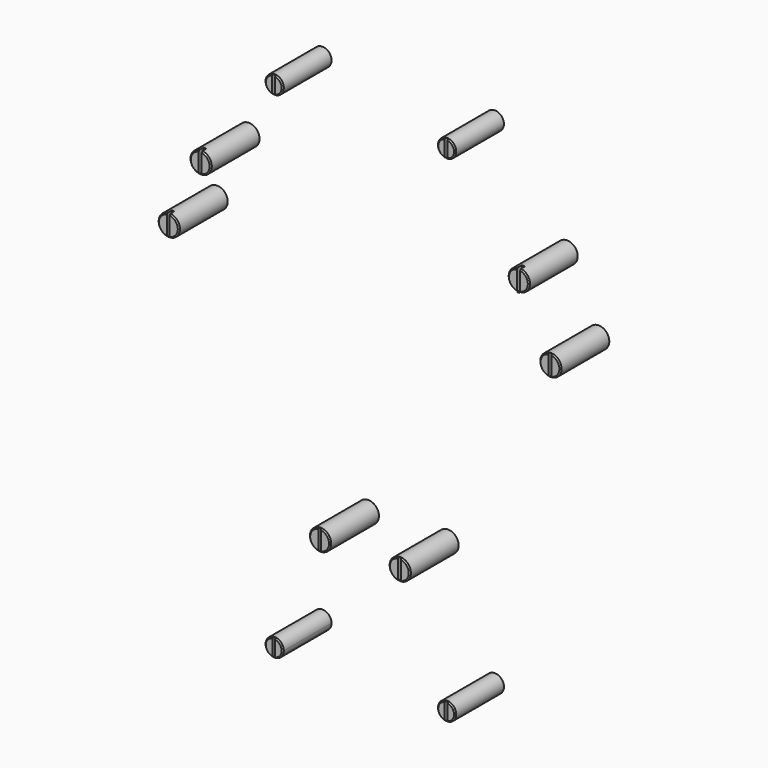
from build123d import *

# Parameters (mm, degrees)
F2_DEPTH      = 25.4
F0_R          = 3.81
F1_R          = 4.445
F4_START      = 22.86
F3_W          = 1.2230351567
F3_H          = 8.8948234916
F3_W_2        = 1.1118501425
F3_W_3        = 1.334220171
F3_H_2        = 8.78364034
F3_W_4        = 1.2230370194
F3_H_3        = 8.5612684488
F3_W_5        = 1.0006669909
F3_H_4        = 8.6724534631
F3_W_6        = 1.0006688535
F3_H_5        = 7.2270408273
F3_W_7        = 1.223038882
F3_W_8        = 1.2295618653
F3_H_6        = 7.377371192
F3_W_9        = 1.3241432607
F3_H_7        = 7.4719488621
F4_DEPTH      = 23.114
F5_4_T2_ANGLE = 279.074624531
F5_4_T4_ANGLE = 119.2903176817
F5_7_C1_SIZE  = 0.508
F5_7_C2_SIZE  = 0.508
F5_8_T2_ANGLE = 278.1597188723
F5_8_T4_ANGLE = 99.7656947124
F5_9_C1_SIZE  = 0.508
F5_9_C2_SIZE  = 0.508


# Not quite as in the source:
# - a fillet or chamfer that OpenCascade refuses, or shapes differently, is made with other operations: its cross-section is extruded or revolved along the edge and cut away or added


with BuildPart() as f2:
    # F0 (on Front) → F2 (new body)
    with BuildSketch(Plane.XZ):
        with BuildLine():
            ThreePointArc((-39.431919848, -111.8159154973), (-35.5624732541, -115.5025815711), (-31.8139005923, -111.6930767894))
            ThreePointArc((-31.8139005923, -111.6930767894), (-35.6853279305, -107.8835720076), (-39.431919848, -111.8159154973))
        make_face()
    extrude(amount=F2_DEPTH)


with BuildPart() as f2b:
    # F0 (on Front) → F2, piece 2 (new body)
    with BuildSketch(Plane.XZ):
        with Locations((36.3284870982, -111.6930693388)):
            Circle(F0_R)
    extrude(amount=F2_DEPTH)


with BuildPart() as f2c:
    # F0 (on Front) → F2, piece 3 (new body)
    with BuildSketch(Plane.XZ):
        with Locations((-35.6239005923, 95.0886905193)):
            Circle(F0_R)
    extrude(amount=F2_DEPTH)


with BuildPart() as f2d:
    # F0 (on Front) → F2, piece 4 (new body)
    with BuildSketch(Plane.XZ):
        with Locations((36.3284870982, 95.0886905193)):
            Circle(F0_R)
    extrude(amount=F2_DEPTH)


with BuildPart() as f2e:
    # F1 (on Front) → F2, piece 5 (new body)
    with BuildSketch(Plane.XZ):
        with Locations((16.7914066574, -65.8985787277)):
            Circle(F1_R)
    extrude(amount=F2_DEPTH)


with BuildPart() as f2f:
    # F1 (on Front) → F2, piece 6 (new body)
    with BuildSketch(Plane.XZ):
        with Locations((-16.4702718891, -65.8985787277)):
            Circle(F1_R)
    extrude(amount=F2_DEPTH)


with BuildPart() as f2g:
    # F1 (on Front) → F2, piece 7 (new body)
    with BuildSketch(Plane.XZ):
        with Locations((-79.6014981537, 29.1146653051)):
            Circle(F1_R)
    extrude(amount=F2_DEPTH)


with BuildPart() as f2h:
    # F1 (on Front) → F2, piece 8 (new body)
    with BuildSketch(Plane.XZ):
        with Locations((-66.3161736801, 56.4890627044)):
            Circle(F1_R)
    extrude(amount=F2_DEPTH)


with BuildPart() as f2i:
    # F1 (on Front) → F2, piece 9 (new body)
    with BuildSketch(Plane.XZ):
        with Locations((66.4782037265, 56.4889616946)):
            Circle(F1_R)
    extrude(amount=F2_DEPTH)


with BuildPart() as f2j:
    # F1 (on Front) → F2, piece 10 (new body)
    with BuildSketch(Plane.XZ):
        with Locations((79.6604069033, 29.5357785845)):
            Circle(F1_R)
    extrude(amount=F2_DEPTH)


with BuildPart() as f4_tool:
    # F3 (on Front) → F4 (new body)
    with BuildSketch(Plane.XZ.offset(F4_START)):
        with Locations((-66.3798488677, 56.613355875)):
            Rectangle(F3_W, F3_H)
        with Locations((-79.6664953232, 29.1505865753)):
            Rectangle(F3_W_2, F3_H)
        with Locations((66.5421783924, 56.5021708608)):
            Rectangle(F3_W_3, F3_H)
        with Locations((79.6620473266, 29.5397331938)):
            Rectangle(F3_W_2, F3_H_2)
        with Locations((16.7867569253, -65.8572539687)):
            Rectangle(F3_W_4, F3_H_3)
        with Locations((-16.4576480165, -65.9128464758)):
            Rectangle(F3_W_5, F3_H_4)
        with Locations((-35.5815198272, -111.6655953228)):
            Rectangle(F3_W_6, F3_H_5)
        with Locations((36.3553669304, -111.7767803371)):
            Rectangle(F3_W_7, F3_H_5)
        with Locations((-35.6421023607, 95.0211137533)):
            Rectangle(F3_W_8, F3_H_6)
        with Locations((36.2872686237, 95.0684025884)):
            Rectangle(F3_W_9, F3_H_7)
    extrude(amount=F4_DEPTH)


with BuildPart() as f2_1:
    add(f2.part)

    # F4: cut by f4_tool
    add(f4_tool.part, mode=Mode.SUBTRACT)

    # F5: chamfer of 0.508 on 1 edges, made by hand

    # F5_s1 → F5_t2 (revolve, cut)
    with BuildSketch(Plane(origin=(3.5622082334, 0, -110.4290151723), x_dir=(0, 1, 0), z_dir=(0.0322411307, 0, -0.9994801196))):
        Polygon((-24.892, -43.016491512), (-25.4, -42.508491512), (-25.4, -43.016491512), align=None)
    revolve(axis=Axis((-35.6239005923, -25.4, -111.6930767894), (0, 1, 0)), mode=Mode.SUBTRACT)


with BuildPart() as f2b_1:
    add(f2b.part)

    # F4: cut by f4_tool
    add(f4_tool.part, mode=Mode.SUBTRACT)

    # F5#2: chamfer of 0.508 on 1 edges, made by hand

    # F5_2_s1 → F5_2_t2 (revolve, cut)
    with BuildSketch(Plane.XY.offset(-111.6930693388)):
        Polygon((40.1384870982, -24.892), (39.6304870982, -25.4), (40.1384870982, -25.4), align=None)
    revolve(axis=Axis((36.3284870982, -25.4, -111.6930693388), (0, -1, 0)), mode=Mode.SUBTRACT)


with BuildPart() as f2c_1:
    add(f2c.part)

    # F4: cut by f4_tool
    add(f4_tool.part, mode=Mode.SUBTRACT)

    # F5#3: chamfer of 0.508 on 1 edges, made by hand

    # F5_3_s1 → F5_3_t2 (revolve, cut)
    with BuildSketch(Plane.XY.offset(95.0886905193)):
        Polygon((-31.8139005923, -24.892), (-32.3219005923, -25.4), (-31.8139005923, -25.4), align=None)
    revolve(axis=Axis((-35.6239005923, -25.4, 95.0886905193), (0, -1, 0)), mode=Mode.SUBTRACT)


with BuildPart() as f2d_1:
    add(f2d.part)

    # F4: cut by f4_tool
    add(f4_tool.part, mode=Mode.SUBTRACT)

    # F5#4: chamfer of 0.508 on 2 edges, made by hand

    # F5_4_s1 → F5_4_t2 (revolve, cut)
    with BuildSketch(Plane.XY.offset(95.0886905193)):
        with BuildLine():
            Line((40.152855508, -24.8776315902), (39.6161186884, -25.4143684098))
            Line((39.6161186884, -25.4143684098), (39.6161186884, -25.4245284098))
            ThreePointArc((39.6161186884, -25.4245284098), (39.8773028933, -25.41016), (40.1384870982, -25.41016))
            Line((40.1384870982, -25.41016), (40.1486470982, -25.4))
            ThreePointArc((40.1486470982, -25.4), (40.1486470982, -25.1388157951), (40.163015508, -24.8776315902))
            Line((40.163015508, -24.8776315902), (40.152855508, -24.8776315902))
        make_face()
    revolve(axis=Axis((36.3284870982, -25.4, 95.0886905193), (0, -1, 0)), revolution_arc=F5_4_T2_ANGLE, mode=Mode.SUBTRACT)

    # F5_4_s3 → F5_4_t4 (revolve, cut)
    with BuildSketch(Plane(origin=(-12.9399105656, 0, 7.2586640976), x_dir=(0, 1, 0), z_dir=(-0.8721519599, 0, 0.4892350752))):
        with BuildLine():
            Line((-24.8776315902, -96.8805895099), (-25.4143684098, -97.4173263294))
            Line((-25.4143684098, -97.4173263294), (-25.4245284098, -97.4173263294))
            ThreePointArc((-25.4245284098, -97.4173263294), (-25.41016, -97.1561421246), (-25.41016, -96.8949579197))
            Line((-25.41016, -96.8949579197), (-25.4, -96.8847979197))
            ThreePointArc((-25.4, -96.8847979197), (-25.1388157951, -96.8847979197), (-24.8776315902, -96.8704295099))
            Line((-24.8776315902, -96.8704295099), (-24.8776315902, -96.8805895099))
        make_face()
    revolve(axis=Axis((36.3284870982, -25.4, 95.0886905193), (0, -1, 0)), revolution_arc=F5_4_T4_ANGLE, mode=Mode.SUBTRACT)


with BuildPart() as f2e_1:
    add(f2e.part)

    # F4: cut by f4_tool
    add(f4_tool.part, mode=Mode.SUBTRACT)

    # F5#5: chamfer of 0.508 on 1 edges, made by hand

    # F5_5_s1 → F5_5_t2 (revolve, cut)
    with BuildSketch(Plane.XY.offset(-65.8985787277)):
        Polygon((21.2364066574, -24.892), (20.7284066574, -25.4), (21.2364066574, -25.4), align=None)
    revolve(axis=Axis((16.7914066574, -25.4, -65.8985787277), (0, -1, 0)), mode=Mode.SUBTRACT)


with BuildPart() as f2f_1:
    add(f2f.part)

    # F4: cut by f4_tool
    add(f4_tool.part, mode=Mode.SUBTRACT)

    # F5#6: chamfer of 0.508 on 1 edges, made by hand

    # F5_6_s1 → F5_6_t2 (revolve, cut)
    with BuildSketch(Plane.XY.offset(-65.8985787277)):
        Polygon((-12.0252718891, -24.892), (-12.5332718891, -25.4), (-12.0252718891, -25.4), align=None)
    revolve(axis=Axis((-16.4702718891, -25.4, -65.8985787277), (0, -1, 0)), mode=Mode.SUBTRACT)


with BuildPart() as f2g_1:
    add(f2g.part)

    # F4: cut by f4_tool
    add(f4_tool.part, mode=Mode.SUBTRACT)

    # F5#7: chamfer of 0.508 on 3 edges, made by hand

    # F5_7_c1
    f5_7_c1_edges = [f2g_1.edges().sort_by_distance(p)[0] for p in [
        (-76.6573079056, -25.4, 25.7845348597),
        (-76.2893840612, -25.4, 32.0791088007),
    ]]
    chamfer(f5_7_c1_edges, length=F5_7_C1_SIZE)

    # F5_7_c2
    f5_7_c2_edges = [f2g_1.edges().sort_by_distance(p)[0] for p in [
        (-84.0464981537, -25.4, 29.1146653051),
    ]]
    chamfer(f5_7_c2_edges, length=F5_7_C2_SIZE)


with BuildPart() as f2h_1:
    add(f2h.part)

    # F4: cut by f4_tool
    add(f4_tool.part, mode=Mode.SUBTRACT)

    # F5#8: chamfer of 0.508 on 2 edges, made by hand

    # F5_8_s1 → F5_8_t2 (revolve, cut)
    with BuildSketch(Plane(origin=(-72.9167311067, 0, 10.4551389996), x_dir=(0, 1, 0), z_dir=(0.9898762599, 0, -0.1419330479))):
        Polygon((-24.892, 50.9497254588), (-25.4, 50.4417254588), (-25.4, 50.9497254588), align=None)
    revolve(axis=Axis((-66.3161736801, -25.4, 56.4890627044), (0, -1, 0)), revolution_arc=F5_8_T2_ANGLE, mode=Mode.SUBTRACT)

    # F5_8_s3 → F5_8_t4 (revolve, cut)
    with BuildSketch(Plane.XY.offset(56.4890627044)):
        Polygon((-61.8711736801, -24.892), (-62.3791736801, -25.4), (-61.8711736801, -25.4), align=None)
    revolve(axis=Axis((-66.3161736801, -25.4, 56.4890627044), (0, -1, 0)), revolution_arc=F5_8_T4_ANGLE, mode=Mode.SUBTRACT)


with BuildPart() as f2i_1:
    add(f2i.part)

    # F4: cut by f4_tool
    add(f4_tool.part, mode=Mode.SUBTRACT)

    # F5#9: chamfer of 0.508 on 3 edges, made by hand

    # F5_9_c1
    f5_9_c1_edges = [f2i_1.edges().sort_by_distance(p)[0] for p in [
        (69.8699360803, -25.4, 53.6159534036),
        (69.8699360803, -25.4, 59.3619699855),
    ]]
    chamfer(f5_9_c1_edges, length=F5_9_C1_SIZE)

    # F5_9_c2
    f5_9_c2_edges = [f2i_1.edges().sort_by_distance(p)[0] for p in [
        (62.0332037265, -25.4, 56.4889616946),
    ]]
    chamfer(f5_9_c2_edges, length=F5_9_C2_SIZE)


with BuildPart() as f2j_1:
    add(f2j.part)

    # F4: cut by f4_tool
    add(f4_tool.part, mode=Mode.SUBTRACT)

    # F5#10: chamfer of 0.508 on 1 edges, made by hand

    # F5_10_s1 → F5_10_t2 (revolve, cut)
    with BuildSketch(Plane.XY.offset(29.5357785845)):
        Polygon((84.1054069033, -24.892), (83.5974069033, -25.4), (84.1054069033, -25.4), align=None)
    revolve(axis=Axis((79.6604069033, -25.4, 29.5357785845), (0, -1, 0)), mode=Mode.SUBTRACT)


solid = Compound([f2_1.part, f2b_1.part, f2c_1.part, f2d_1.part, f2e_1.part, f2f_1.part, f2g_1.part, f2h_1.part, f2i_1.part, f2j_1.part])
